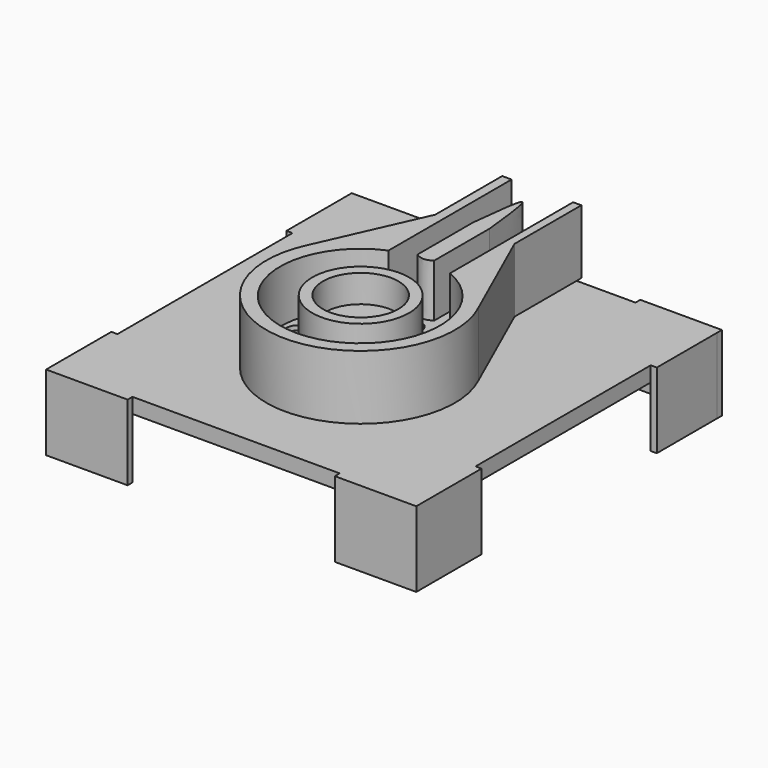
from build123d import *

# Parameters (mm, degrees)
F0_R     = 1.9095863366
F0_R_2   = 1.9061403528
F0_R_3   = 8.144338214
F0_R_4   = 1.8999548266
F0_R_5   = 1.9002502649
F0_R_6   = 6.35
F1_DEPTH = 1.905
F2_DEPTH = 10.795
F3_R     = 5.969
F5_DEPTH = 6.35
F3_R_2   = 13.208
F6_DEPTH = 1.143
F4_R     = 13.329687055
F4_R_2   = 6.096
F7_DEPTH = 1.143
F8_DEPTH = 2.54
F9_DEPTH = 12.7


with BuildPart() as f1:
    # F0 (on Top) → F1 (new body)
    with BuildSketch(Plane.XY):
        with BuildLine():
            Line((-6.6588919425, 24.025004246), (-14.3305402873, 6.8301713064))
            ThreePointArc((-14.3305402873, 6.8301713064), (0.000639197, -15.8749999871), (14.3299902157, 6.8313253047))
            Line((14.3299902157, 6.8313253047), (6.6590019569, 24.045052064))
            Line((6.6590019569, 24.045052064), (6.6590019569, 38.1))
            Line((6.6590019569, 38.1), (5.2753846154, 38.1))
            Line((5.2753846154, 38.1), (5.2753846154, 12.192))
            ThreePointArc((5.2753846154, 12.192), (0.0976923077, -13.6964615385), (-5.08, 12.192))
            Line((-5.08, 12.192), (-5.08, 38.1))
            Line((-5.08, 38.1), (-6.6588919425, 38.1))
            Line((-6.6588919425, 38.1), (-6.6588919425, 24.025004246))
        make_face()
        with BuildLine():
            Line((5.2753846154, 38.1), (-5.08, 38.1))
            Line((-5.08, 38.1), (-5.08, 12.192))
            ThreePointArc((-5.08, 12.192), (0.0976923077, -13.6964615385), (5.2753846154, 12.192))
            Line((5.2753846154, 12.192), (5.2753846154, 38.1))
        make_face()
        with Locations((0, -10.9124137089)):
            Circle(F0_R, mode=Mode.SUBTRACT)
        with Locations((-10.5649987236, 0)):
            Circle(F0_R_2, mode=Mode.SUBTRACT)
        Circle(F0_R_3, mode=Mode.SUBTRACT)
        with Locations((0, 10.4045402259)):
            Circle(F0_R_4, mode=Mode.SUBTRACT)
        with Locations((10.7626086032, 0.0003860946)):
            Circle(F0_R_5, mode=Mode.SUBTRACT)
        with BuildLine():
            add(Edge.make_bspline(
                [(-1.397, 13.6617869139), (-0.9313333333, 13.4348934569), (0, 12.9811065431), (0.9313333333, 13.4348934569), (1.397, 13.6617869139)],
                knots=[0, 0, 0, 0, 0.5, 1, 1, 1, 1], degree=3))
            Line((-1.397, 13.6617869139), (-1.397, 17.2657109797))
            Line((-1.397, 17.2657109797), (-1.397, 25.3996907175))
            add(Edge.make_bspline(
                [(-1.397, 25.3996907175), (-0.9313529757, 29.6944177327), (-0.0001374736, 38.2831473186), (0.9313136976, 29.69591761), (1.397, 25.4026649147)],
                knots=[0, 0, 0, 0, 0.5000421741, 1, 1, 1, 1], degree=3))
            Line((1.397, 25.4026649147), (1.397, 17.2657109797))
            Line((1.397, 17.2657109797), (1.397, 13.6617869139))
        make_face(mode=Mode.SUBTRACT)
        with BuildLine():
            Line((-1.397, 17.2657109797), (-1.397, 13.6617869139))
            add(Edge.make_bspline(
                [(-1.397, 13.6617869139), (-0.9313333333, 13.4348934569), (0, 12.9811065431), (0.9313333333, 13.4348934569), (1.397, 13.6617869139)],
                knots=[0, 0, 0, 0, 0.5, 1, 1, 1, 1], degree=3))
            Line((1.397, 13.6617869139), (1.397, 17.2657109797))
            Line((1.397, 17.2657109797), (1.397, 25.4026649147))
            add(Edge.make_bspline(
                [(-1.397, 25.3996907175), (-0.9313529757, 29.6944177327), (-0.0001374736, 38.2831473186), (0.9313136976, 29.69591761), (1.397, 25.4026649147)],
                knots=[0, 0, 0, 0, 0.5000421741, 1, 1, 1, 1], degree=3))
            Line((-1.397, 25.3996907175), (-1.397, 17.2657109797))
        make_face()
        Circle(F0_R_3)
        Circle(F0_R_6, mode=Mode.SUBTRACT)
    extrude(amount=F1_DEPTH)

    # F0 (on Top) → F2 (join)
    with BuildSketch(Plane.XY):
        Circle(F0_R_3)
        Circle(F0_R_6, mode=Mode.SUBTRACT)
        with BuildLine():
            Line((-6.6588919425, 24.025004246), (-14.3305402873, 6.8301713064))
            ThreePointArc((-14.3305402873, 6.8301713064), (0.000639197, -15.8749999871), (14.3299902157, 6.8313253047))
            Line((14.3299902157, 6.8313253047), (6.6590019569, 24.045052064))
            Line((6.6590019569, 24.045052064), (6.6590019569, 38.1))
            Line((6.6590019569, 38.1), (5.2753846154, 38.1))
            Line((5.2753846154, 38.1), (5.2753846154, 12.192))
            ThreePointArc((5.2753846154, 12.192), (0.0976923077, -13.6964615385), (-5.08, 12.192))
            Line((-5.08, 12.192), (-5.08, 38.1))
            Line((-5.08, 38.1), (-6.6588919425, 38.1))
            Line((-6.6588919425, 38.1), (-6.6588919425, 24.025004246))
        make_face()
        with BuildLine():
            Line((-1.397, 17.2657109797), (-1.397, 13.6617869139))
            add(Edge.make_bspline(
                [(-1.397, 13.6617869139), (-0.9313333333, 13.4348934569), (0, 12.9811065431), (0.9313333333, 13.4348934569), (1.397, 13.6617869139)],
                knots=[0, 0, 0, 0, 0.5, 1, 1, 1, 1], degree=3))
            Line((1.397, 13.6617869139), (1.397, 17.2657109797))
            Line((1.397, 17.2657109797), (1.397, 25.4026649147))
            add(Edge.make_bspline(
                [(-1.397, 25.3996907175), (-0.9313529757, 29.6944177327), (-0.0001374736, 38.2831473186), (0.9313136976, 29.69591761), (1.397, 25.4026649147)],
                knots=[0, 0, 0, 0, 0.5000421741, 1, 1, 1, 1], degree=3))
            Line((-1.397, 25.3996907175), (-1.397, 17.2657109797))
        make_face()
    extrude(amount=F2_DEPTH)


with BuildPart() as f5:
    # F3 (on Top) → F5 (new body)
    with BuildSketch(Plane.XY):
        Circle(F3_R)
    extrude(amount=F5_DEPTH)

    # F3 (on Top) → F6 (join)
    with BuildSketch(Plane.XY):
        Circle(F3_R_2)
        Circle(F3_R, mode=Mode.SUBTRACT)
    extrude(amount=F6_DEPTH)


with BuildPart() as f7:
    # F4 (on Top) → F7 (new body)
    with BuildSketch(Plane.XY):
        Polygon((-30.9983175248, -12.4335922301), (-30.9983175248, -25.1362901181), (-18.3023493737, -25.1362901181), (0, -25.1362901181), (16.5724009275, -25.1362901181), (29.2792506516, -25.1362901181), (29.2792506516, -12.4335922301), (29.2792506516, 24.4187787175), (29.2792506516, 37.1073037386), (16.5714547038, 37.1073037386), (-18.2970520109, 37.1073037386), (-30.9983175248, 37.1073037386), (-30.9983175248, 24.4006793946), (-30.9983175248, 0), align=None)
        Circle(F4_R, mode=Mode.SUBTRACT)
        Circle(F4_R)
        Circle(F4_R_2, mode=Mode.SUBTRACT)
        Polygon((29.2792506516, -25.1362901181), (16.5724009275, -25.1362901181), (16.5724009275, -26.1582173407), (29.2792506516, -26.1582173407), (30.2841644734, -26.1582173407), (30.2841644734, -25.1362901181), (30.2841644734, -12.4335922301), (29.2792506516, -12.4335922301), align=None)
    extrude(amount=-F7_DEPTH)

    # F4 (on Top) → F8 (join)
    with BuildSketch(Plane.XY):
        Polygon((-30.9983175248, -12.4335922301), (-30.9983175248, -25.1362901181), (-18.3023493737, -25.1362901181), (0, -25.1362901181), (16.5724009275, -25.1362901181), (29.2792506516, -25.1362901181), (29.2792506516, -12.4335922301), (29.2792506516, 24.4187787175), (29.2792506516, 37.1073037386), (16.5714547038, 37.1073037386), (-18.2970520109, 37.1073037386), (-30.9983175248, 37.1073037386), (-30.9983175248, 24.4006793946), (-30.9983175248, 0), align=None)
        Circle(F4_R, mode=Mode.SUBTRACT)
        Polygon((-18.3023493737, -25.1362901181), (-30.9983175248, -25.1362901181), (-30.9983175248, -12.4335922301), (-32.0252366364, -12.4335922301), (-32.0252366364, -25.1362901181), (-32.0252366364, -26.1582173407), (-30.9983175248, -26.1582173407), (-18.3023493737, -26.1582173407), align=None)
        Polygon((29.2792506516, -25.1362901181), (16.5724009275, -25.1362901181), (16.5724009275, -26.1582173407), (29.2792506516, -26.1582173407), (30.2841644734, -26.1582173407), (30.2841644734, -25.1362901181), (30.2841644734, -12.4335922301), (29.2792506516, -12.4335922301), align=None)
        Polygon((-32.0145189762, 24.4006793946), (-30.9983175248, 24.4006793946), (-30.9983175248, 37.1073037386), (-18.2970520109, 37.1073037386), (-18.2970520109, 38.1312929094), (-30.9983175248, 38.1312929094), (-32.0145189762, 38.1312929094), (-32.0145189762, 37.1073037386), align=None)
        Polygon((29.2792506516, 37.1073037386), (29.2792506516, 24.4187787175), (30.3034484386, 24.4187787175), (30.3034484386, 37.1073037386), (30.3062088788, 38.1182320416), (29.2792506516, 38.1182320416), (16.5714547038, 38.1182320416), (16.5714547038, 37.1073037386), align=None)
    extrude(amount=-F8_DEPTH)

    # F4 (on Top) → F9 (join)
    with BuildSketch(Plane.XY):
        Polygon((-32.0145189762, 24.4006793946), (-30.9983175248, 24.4006793946), (-30.9983175248, 37.1073037386), (-18.2970520109, 37.1073037386), (-18.2970520109, 38.1312929094), (-30.9983175248, 38.1312929094), (-32.0145189762, 38.1312929094), (-32.0145189762, 37.1073037386), align=None)
        Polygon((-18.3023493737, -25.1362901181), (-30.9983175248, -25.1362901181), (-30.9983175248, -12.4335922301), (-32.0252366364, -12.4335922301), (-32.0252366364, -25.1362901181), (-32.0252366364, -26.1582173407), (-30.9983175248, -26.1582173407), (-18.3023493737, -26.1582173407), align=None)
        Polygon((29.2792506516, -25.1362901181), (16.5724009275, -25.1362901181), (16.5724009275, -26.1582173407), (29.2792506516, -26.1582173407), (30.2841644734, -26.1582173407), (30.2841644734, -25.1362901181), (30.2841644734, -12.4335922301), (29.2792506516, -12.4335922301), align=None)
        Polygon((29.2792506516, 37.1073037386), (29.2792506516, 24.4187787175), (30.3034484386, 24.4187787175), (30.3034484386, 37.1073037386), (30.3062088788, 38.1182320416), (29.2792506516, 38.1182320416), (16.5714547038, 38.1182320416), (16.5714547038, 37.1073037386), align=None)
    extrude(amount=-F9_DEPTH)


solid = Compound([f1.part, f5.part, f7.part])
